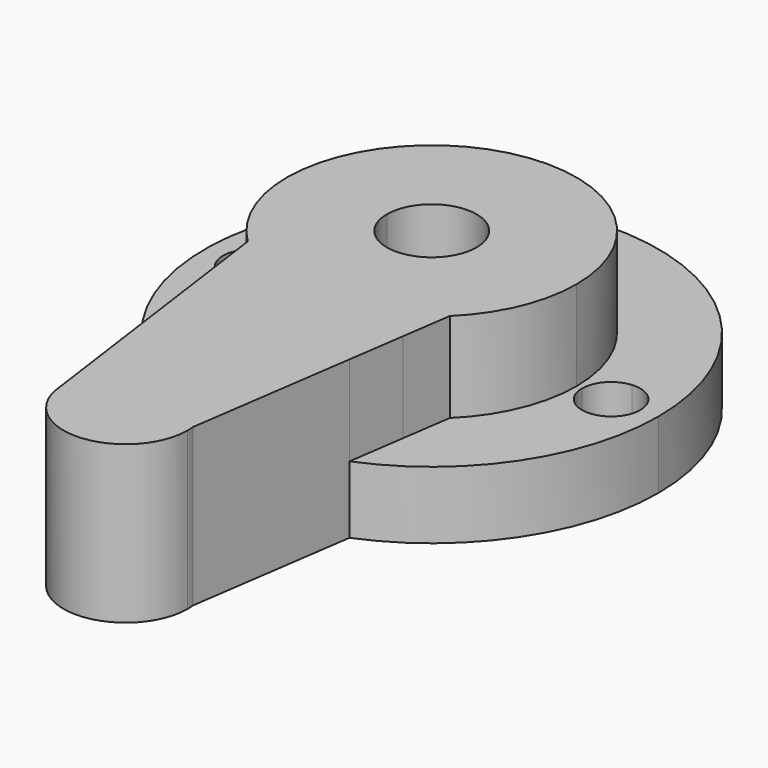
from build123d import *

# Parameters (mm, degrees)
F1_DEPTH = 7
F2_DEPTH = 3
F3_DEPTH = 3


# Not quite as in the source:
# - a feature names something its author has since deleted; it is built from what else it names


with BuildPart() as f1:
    # F0 (on Top) → F1 (new body)
    with BuildSketch(Plane.XY):
        with BuildLine():
            Line((-1.1851356201, 23.1923339907), (-5.6851356201, 23.1923339907))
            ThreePointArc((-5.6851356201, 23.1923339907), (-3.6139055058, 21.83796352), (-1.1851356201, 21.3632105309))
            Line((-1.1851356201, 21.3632105309), (-1.1851356201, 23.1923339907))
        make_face()
        with BuildLine():
            ThreePointArc((-1.1851356201, 21.3632105309), (1.2436342657, 21.83796352), (3.3148643799, 23.1923339907))
            Line((3.3148643799, 23.1923339907), (-1.1851356201, 23.1923339907))
            Line((-1.1851356201, 23.1923339907), (-1.1851356201, 21.3632105309))
        make_face()
        with BuildLine():
            ThreePointArc((-7.6351356201, 27.8132105309), (-7.1276729569, 25.3054725063), (-5.6851356201, 23.1923339907))
            Line((-5.6851356201, 23.1923339907), (-1.1851356201, 23.1923339907))
            Line((-1.1851356201, 23.1923339907), (-1.1851356201, 25.8132105309))
            ThreePointArc((-1.1851356201, 25.8132105309), (-2.5993491824, 26.3989969686), (-3.1851356201, 27.8132105309))
            Line((-3.1851356201, 27.8132105309), (-7.6351356201, 27.8132105309))
        make_face()
        with BuildLine():
            Line((-1.1851356201, 23.1923339907), (3.3148643799, 23.1923339907))
            ThreePointArc((3.3148643799, 23.1923339907), (4.7574017168, 25.3054725063), (5.2648643799, 27.8132105309))
            Line((5.2648643799, 27.8132105309), (0.8148643799, 27.8132105309))
            ThreePointArc((0.8148643799, 27.8132105309), (0.2290779423, 26.3989969686), (-1.1851356201, 25.8132105309))
            Line((-1.1851356201, 25.8132105309), (-1.1851356201, 23.1923339907))
        make_face()
        with BuildLine():
            Line((-5.0348369716, 18.4756626995), (-3.9452707751, 10.572946599))
            ThreePointArc((-3.9452707751, 10.572946599), (-3.2076275018, 12.6510857986), (-1.1851356201, 13.5298956301))
            Line((-1.1851356201, 13.5298956301), (-1.1851356201, 17.7132105309))
            ThreePointArc((-1.18513562, 17.7132105309), (-3.1473750171, 17.9056570212), (-5.0348369716, 18.4756626995))
        make_face()
        with BuildLine():
            ThreePointArc((-3.9452707751, 10.572946599), (-1.0899472994, 7.9981634027), (1.5815494791, 10.7632105309))
            ThreePointArc((1.5815494791, 10.7632105309), (1.5769058667, 10.923439316), (1.562990617, 11.0831302441))
            ThreePointArc((1.562990617, 11.0831302441), (0.6546237847, 12.8295676566), (-1.1851356201, 13.5298956301))
            ThreePointArc((-1.1851356201, 13.5298956301), (-3.2076275018, 12.6510857986), (-3.9452707751, 10.572946599))
        make_face()
        with BuildLine():
            Line((-5.3833250343, 21.0032761963), (-5.0348369716, 18.4756626995))
            ThreePointArc((-5.0348369716, 18.4756626995), (-3.1473750171, 17.9056570212), (-1.18513562, 17.7132105309))
            Line((-1.1851356201, 17.7132105309), (-1.1851356201, 19.8132105309))
            ThreePointArc((-1.1851356201, 19.8132105309), (-3.3669382375, 20.1164750321), (-5.3833250343, 21.0032761963))
        make_face()
        with BuildLine():
            Line((-5.6851356201, 23.1923339907), (-5.3833250343, 21.0032761963))
            ThreePointArc((-5.3833250343, 21.0032761963), (-3.3669382375, 20.1164750321), (-1.1851356201, 19.8132105309))
            Line((-1.1851356201, 19.8132105309), (-1.1851356201, 21.3632105309))
            ThreePointArc((-1.1851356201, 21.3632105309), (-3.6139055058, 21.83796352), (-5.6851356201, 23.1923339907))
        make_face()
        with BuildLine():
            ThreePointArc((-1.1851356201, 13.5298956301), (0.6546237847, 12.8295676566), (1.562990617, 11.0831302441))
            Line((1.562990617, 11.0831302441), (2.630466448, 18.461676921))
            ThreePointArc((2.630466448, 18.461676921), (0.7590236506, 17.9020933018), (-1.18513562, 17.7132105309))
            Line((-1.1851356201, 17.7132105309), (-1.1851356201, 13.5298956301))
        make_face()
        with BuildLine():
            ThreePointArc((-1.18513562, 17.7132105309), (0.7590236506, 17.9020933018), (2.630466448, 18.461676921))
            Line((2.630466448, 18.461676921), (2.9967135721, 20.993229788))
            ThreePointArc((2.9967135721, 20.993229788), (0.9874382057, 20.1138649112), (-1.1851356201, 19.8132105309))
            Line((-1.1851356201, 19.8132105309), (-1.1851356201, 17.7132105309))
        make_face()
        with BuildLine():
            ThreePointArc((-1.1851356201, 19.8132105309), (0.9874382057, 20.1138649112), (2.9967135721, 20.993229788))
            Line((2.9967135721, 20.993229788), (3.3148643799, 23.1923339907))
            ThreePointArc((3.3148643799, 23.1923339907), (1.2436342657, 21.83796352), (-1.1851356201, 21.3632105309))
            Line((-1.1851356201, 21.3632105309), (-1.1851356201, 19.8132105309))
        make_face()
        with BuildLine():
            Line((0.8148643799, 27.8132105309), (5.2648643799, 27.8132105309))
            ThreePointArc((5.2648643799, 27.8132105309), (-1.1851356201, 34.2632105309), (-7.6351356201, 27.8132105309))
            Line((-7.6351356201, 27.8132105309), (-3.1851356201, 27.8132105309))
            ThreePointArc((-3.1851356201, 27.8132105309), (-1.1851356201, 29.8132105309), (0.8148643799, 27.8132105309))
        make_face()
    extrude(amount=F1_DEPTH)

    # F0 (on Top) → F2 (join)
    with BuildSketch(Plane.XY):
        with BuildLine():
            Line((2.9967135721, 20.993229788), (2.630466448, 18.461676921))
            ThreePointArc((2.630466448, 18.461676921), (7.1978107858, 22.179720533), (8.9148643799, 27.8132105309))
            ThreePointArc((8.9148643799, 27.8132105309), (-6.8033211078, 36.2064215866), (-5.0348369716, 18.4756626995))
            Line((-5.0348369716, 18.4756626995), (-5.3833250343, 21.0032761963))
            ThreePointArc((-5.3833250343, 21.0032761963), (-7.8303759033, 23.3589113068), (-9.0795106201, 26.5175086519))
            ThreePointArc((-9.0795106201, 26.5175086519), (-10.4851356201, 27.8132105309), (-9.0795106201, 29.10891241))
            ThreePointArc((-9.0795106201, 29.10891241), (-6.8419898695, 33.4700647804), (-2.4808374991, 35.7075855309))
            ThreePointArc((-2.4808374991, 35.7075855309), (-1.237991827, 37.1121355562), (0.1148643799, 35.8132105309))
            ThreePointArc((0.1148643799, 35.8132105309), (0.1137894053, 35.7603543239), (0.110566259, 35.7075855309))
            ThreePointArc((0.110566259, 35.7075855309), (4.4752873931, 33.4664937639), (6.7108684576, 29.0989475203))
            ThreePointArc((6.7108684576, 29.0989475203), (7.6965647575, 28.7584108036), (8.1148580079, 27.803113359))
            ThreePointArc((8.1148580079, 27.803113359), (7.6953583299, 26.8467038322), (6.7075977264, 26.5075458262))
            ThreePointArc((6.7075977264, 26.5075458262), (5.4519425182, 23.3467584953), (2.9967135721, 20.993229788))
        make_face()
        with BuildLine():
            ThreePointArc((-9.0795106201, 26.5175086519), (-7.8303759033, 23.3589113068), (-5.3833250343, 21.0032761963))
            Line((-5.3833250343, 21.0032761963), (-5.6851356201, 23.1923339907))
            ThreePointArc((-5.6851356201, 23.1923339907), (-7.1276729569, 25.3054725063), (-7.6351356201, 27.8132105309))
            Line((-7.6351356201, 27.8132105309), (-7.8851356201, 27.8132105309))
            ThreePointArc((-7.8851356201, 27.8132105309), (-8.229281944, 26.9321068197), (-9.0795106201, 26.5175086519))
        make_face()
    extrude(amount=F2_DEPTH)

    # F0 (on Top) → F3 (join)
    with BuildSketch(Plane.XY):
        with BuildLine():
            Line((3.3148643799, 23.1923339907), (2.9967135721, 20.993229788))
            ThreePointArc((2.9967135721, 20.993229788), (5.4519425182, 23.3467584953), (6.7075977264, 26.5075458262))
            ThreePointArc((6.7075977264, 26.5075458262), (5.8555856645, 26.9257328422), (5.5148855907, 27.81158181))
            Line((5.5148855907, 27.81158181), (5.2648643799, 27.8132105309))
            ThreePointArc((5.2648643799, 27.8132105309), (4.7574017168, 25.3054725063), (3.3148643799, 23.1923339907))
        make_face()
        with BuildLine():
            ThreePointArc((-7.6351356201, 27.8132105309), (-1.1851356201, 34.2632105309), (5.2648643799, 27.8132105309))
            Line((5.2648643799, 27.8132105309), (5.5148855907, 27.81158181))
            ThreePointArc((5.5148855907, 27.81158181), (5.8624374498, 28.6879269442), (6.7108684576, 29.0989475203))
            ThreePointArc((6.7108684576, 29.0989475203), (4.4752873931, 33.4664937639), (0.110566259, 35.7075855309))
            ThreePointArc((0.110566259, 35.7075855309), (-1.1851356201, 34.5132105309), (-2.4808374991, 35.7075855309))
            ThreePointArc((-2.4808374991, 35.7075855309), (-6.8419898695, 33.4700647804), (-9.0795106201, 29.10891241))
            ThreePointArc((-9.0795106201, 29.10891241), (-8.229281944, 28.6943142422), (-7.8851356201, 27.8132105309))
            Line((-7.8851356201, 27.8132105309), (-7.6351356201, 27.8132105309))
        make_face()
    extrude(amount=F3_DEPTH)


solid = f1.part
